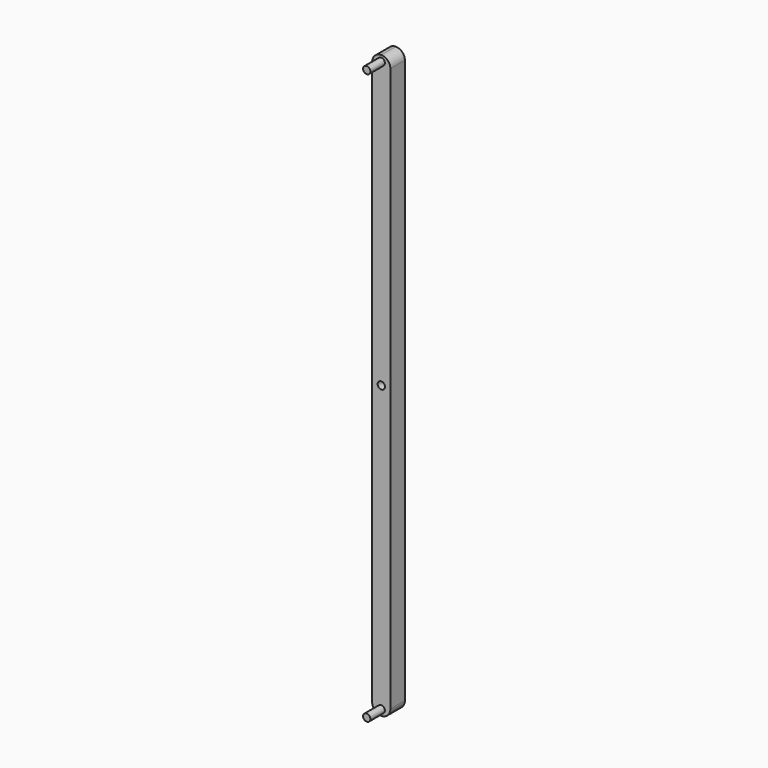
from build123d import *

# Parameters (mm, degrees)
F0_W     = 25
F0_H     = 800
F1_DEPTH = 25
F2_R     = 5
F3_DEPTH = 25
F4_R     = 5
F5_DEPTH = 25
F6_R     = 12.49999
F7_R     = 12.49999


# Not quite as in the source:
# - a fillet or chamfer is up to 0.001 mm smaller than in the source, because OpenCascade refuses the exact size
# - a pattern or mirror of a feature is missing from the dataset's text; its kind, count and spacing are read off the source's solid


with BuildPart() as f1:
    # F0 (on Front) → F1 (new body)
    with BuildSketch(Plane.XZ):
        Rectangle(F0_W, F0_H)
    extrude(amount=F1_DEPTH)

    # F2 (on face) → F3 (join)
    with BuildSketch(Plane.XZ.offset(25)):
        with Locations((0, 391.8639719486)):
            Circle(F2_R)
    f3 = extrude(amount=F3_DEPTH)

    # F3_copies: F3 across plane
    add(f3.mirror(Plane(origin=(0, 0, 0), x_dir=(-1, 0, 0), z_dir=(0, 0, -1))))

    # F4 (on face) → F5 (cut)
    with BuildSketch(Plane.XZ.offset(25)):
        Circle(F4_R)
    extrude(amount=-F5_DEPTH, mode=Mode.SUBTRACT)

    # F6 (radius 12.5 in the source; OpenCascade refuses exactly that, so slightly less here)
    f6_edges = [f1.edges().sort_by_distance(p)[0] for p in [
        (-12.5, -12.5, 400),
        (12.5, -12.5, 400),
    ]]
    fillet(f6_edges, radius=F6_R)

    # F7 (radius 12.5 in the source; OpenCascade refuses exactly that, so slightly less here)
    f7_edges = [f1.edges().sort_by_distance(p)[0] for p in [
        (12.5, -12.5, -400),
        (-12.5, -12.5, -400),
    ]]
    fillet(f7_edges, radius=F7_R)


solid = f1.part
